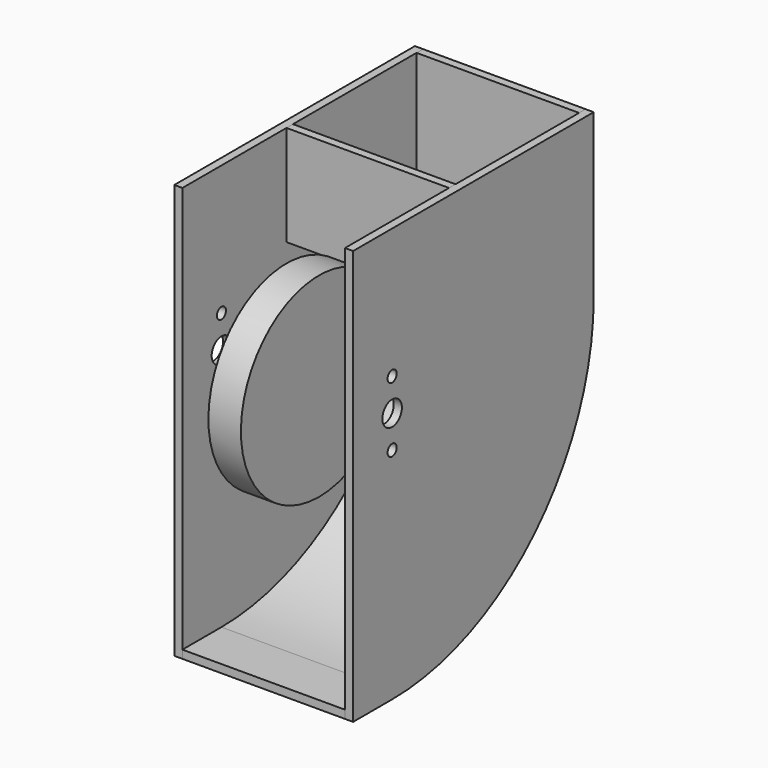
from build123d import *

# Parameters (mm, degrees)
F1_DEPTH      = 63.5
F1_DEPTH_BACK = 63.5
F2_DEPTH      = 12.7
F2_DEPTH_BACK = 12.7
F4_DEPTH      = 6.35
F5_R          = 4.445
F5_R_2        = 9.525
F6_DEPTH      = 25.4
F9_W          = 6.3508271281
F9_H          = 78.5272554297
F10_DEPTH     = 127
F11_DEPTH     = 38.1


with BuildPart() as f1:
    # F0 (on Right) → F1 (new body, two sides)
    with BuildSketch(Plane.YZ) as f1_sk:
        with BuildLine():
            Line((196.8499965305, 0), (190.5, 0))
            ThreePointArc((190.5, 0), (134.703841816, -134.703841816), (0, -190.5))
            Line((0, -190.5), (0, -196.8499965305))
            ThreePointArc((0, -196.8499965305), (139.1939674233, -139.1939674233), (196.8499965305, 0))
        make_face()
        with BuildLine():
            ThreePointArc((190.5, 49.5950716712), (195.2560440462, 24.99996795), (196.8499965305, 0))
            Line((196.8499965305, 0), (196.8499965305, 127))
            Line((196.8499965305, 127), (190.5, 127))
            Line((190.5, 127), (190.5, 49.5950716712))
        make_face()
        with BuildLine():
            Line((190.5, 49.5950716712), (190.5, 0))
            Line((190.5, 0), (196.8499965305, 0))
            ThreePointArc((196.8499965305, 0), (195.2560440462, 24.99996795), (190.5, 49.5950716712))
        make_face()
    extrude(amount=F1_DEPTH)
    extrude(f1_sk.sketch, amount=-F1_DEPTH_BACK)

    # F11 (add, through all): a face of the model
    f11_faces = [f1.faces().sort_by_distance(p)[0] for p in [
        (0, 0, -193.6749982653),
    ]]
    extrude(f11_faces, amount=F11_DEPTH)


with BuildPart() as f2:
    # F0 (on Right) → F2 (new body, two sides)
    with BuildSketch(Plane.YZ) as f2_sk:
        with BuildLine():
            Line((0, 0), (76.2, 0))
            ThreePointArc((76.2, 0), (-53.8815367264, 53.8815367264), (0, -76.2))
            Line((0, -76.2), (0, 0))
        make_face()
        with BuildLine():
            ThreePointArc((0, -76.2), (53.8815367264, -53.8815367264), (76.2, 0))
            Line((76.2, 0), (0, 0))
            Line((0, 0), (0, -76.2))
        make_face()
    extrude(amount=F2_DEPTH)
    extrude(f2_sk.sketch, amount=-F2_DEPTH_BACK)


with BuildPart() as f4:
    # F3 (on face) → F4 (new body)
    with BuildSketch(Plane(origin=(-63.5, 0, 0), x_dir=(0, -1, 0), z_dir=(-1, 0, 0))):
        with BuildLine():
            Line((-196.8499965305, 127), (-196.8499965305, 0))
            ThreePointArc((-196.8499965305, 0), (-139.1939674233, -139.1939674233), (0, -196.8499965305))
            Line((0, -196.8499965305), (0, -190.5))
            ThreePointArc((0, -190.5), (-134.703841816, -134.703841816), (-190.5, 0))
            Line((-190.5, 0), (-190.5, 127))
            Line((-190.5, 127), (-196.8499965305, 127))
        make_face()
        with BuildLine():
            Line((0, -190.5), (0, -196.8499965305))
            Line((0, -196.8499965305), (38.1, -196.8499965305))
            Line((38.1, -196.8499965305), (38.1, -65.9911357684))
            ThreePointArc((38.1, -65.9911357684), (-76.2, 0), (38.1, 65.9911357684))
            Line((38.1, 65.9911357684), (38.1, 127))
            Line((38.1, 127), (-190.5, 127))
            Line((-190.5, 127), (-190.5, 0))
            ThreePointArc((-190.5, 0), (-134.703841816, -134.703841816), (0, -190.5))
        make_face()
        with BuildLine():
            ThreePointArc((38.1, 65.9911357684), (-76.2, 0), (38.1, -65.9911357684))
            Line((38.1, -65.9911357684), (38.1, 0))
            Line((38.1, 0), (38.1, 65.9911357684))
        make_face()
    extrude(amount=F4_DEPTH)

    # F5 (on face) → F6 (cut)
    with BuildSketch(Plane(origin=(-69.85, 0, 0), x_dir=(0, -1, 0), z_dir=(-1, 0, 0))):
        with Locations((0, 25.4)):
            Circle(F5_R)
        Circle(F5_R_2)
        with Locations((0, -25.4)):
            Circle(F5_R)
    extrude(amount=-F6_DEPTH, mode=Mode.SUBTRACT)


with BuildPart() as f8_1:
    # F8: copy of F4
    add(f4.part.moved(Location((133.35, 0, 0))))


with BuildPart() as f10:
    # F9 (on face) → F10 (new body, through all)
    with BuildSketch(Plane.YZ.offset(-63.5)):
        with Locations((66.6743457587, 87.7363722852)):
            Rectangle(F9_W, F9_H)
    extrude(amount=F10_DEPTH)


solid = Compound([f1.part, f2.part, f4.part, f8_1.part, f10.part])
